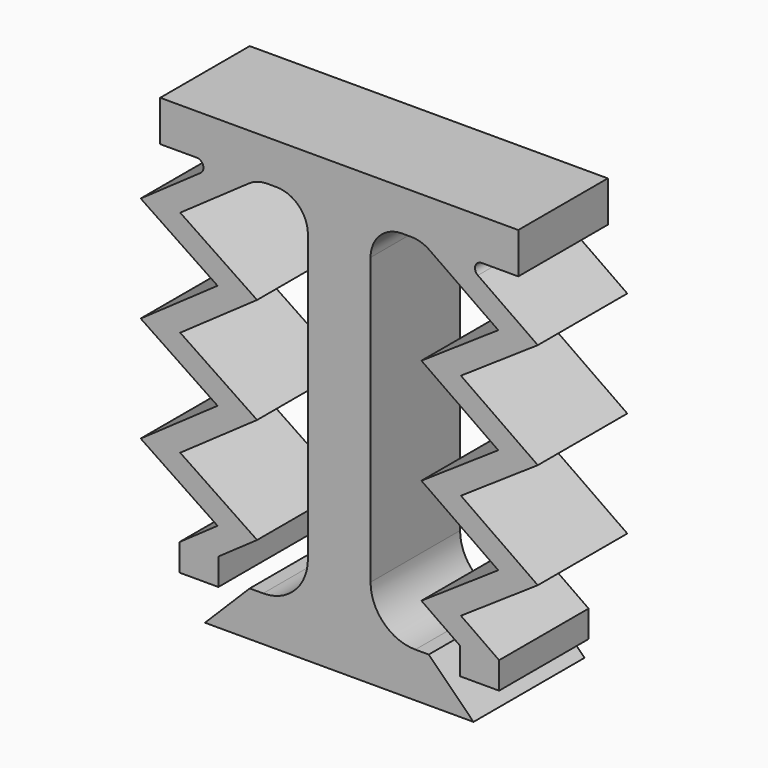
from build123d import *

# Parameters (mm, degrees)
F0_W     = 0.8717233978
F0_H     = 0.6
F1_DEPTH = 2.5
F2_DEPTH = 0.6
F4_SIZE  = 0.59999
F5_R     = 0.7
F6_R     = 1
F7_R     = 0.15


# Not quite as in the source:
# - a fillet or chamfer is up to 0.001 mm smaller than in the source, because OpenCascade refuses the exact size


with BuildPart() as f1:
    # F0 (on Front) → F1 (new body)
    with BuildSketch(Plane.XZ):
        Polygon((0, 1), (0, 0), (3, 0), (2, 1), (0.7, 1), align=None)
        Polygon((2.7075850967, 9.087372576), (1.8358616989, 9.087372576), (3.5531366706, 7.8849236956), (1.8358616989, 6.7266071015), (3.5531366706, 5.5241582211), (1.8358616989, 4.365841627), (3.5531366706, 3.1633927466), (1.8358616989, 2.0050761525), (2.7, 1.4), (3.5717233978, 1.4), (2.7185867272, 1.9973727279), (4.4358616989, 3.155689322), (2.7185867272, 4.3581382024), (4.4358616989, 5.5164547965), (2.7185867272, 6.7189036769), (4.4358616989, 7.877220271), align=None)
        with Locations((3.1358616989, 1.1)):
            Rectangle(F0_W, F0_H)
        Polygon((0, 9), (0, 1), (0.7, 1), (0.7, 9.087372576), (1.8358616989, 9.087372576), (2.7075850967, 9.087372576), (4, 9.087372576), (4, 10), (0, 10), align=None)
    extrude(amount=F1_DEPTH)

    # F0 (on Front) → F2 (join)
    with BuildSketch(Plane.XZ):
        Polygon((0, 1), (0, 0), (3, 0), (2, 1), (0.7, 1), align=None)
    extrude(amount=-F2_DEPTH)

    # F3: F1 across face


with BuildPart() as f1_1:
    add(f1.part)
    add(f1.part.mirror(Plane(origin=(0, -1.213671875, 4.89453125), x_dir=(0, -1, 0), z_dir=(-1, 0, 0))))

    # F4 (size 0.6 in the source; OpenCascade refuses exactly that, so slightly less here)
    f4_edges = [f1_1.edges().sort_by_distance(p)[0] for p in [
        (0, 0.6, 1),
    ]]
    chamfer(f4_edges, length=F4_SIZE)

    # F5
    f5_edges = [f1_1.edges().sort_by_distance(p)[0] for p in [
        (0.7, -1.25, 9.087373),
        (-0.7, -1.25, 9.087373),
        (1.835862, -1.25, 9.087373),
        (-1.835862, -1.25, 9.087373),
    ]]
    fillet(f5_edges, radius=F5_R)

    # F6
    f6_edges = [f1_1.edges().sort_by_distance(p)[0] for p in [
        (0.7, -1.25, 1),
        (-0.7, -1.25, 1),
    ]]
    fillet(f6_edges, radius=F6_R)

    # F7
    f7_edges = [f1_1.edges().sort_by_distance(p)[0] for p in [
        (2.707585, -1.25, 9.087373),
        (-2.707585, -1.25, 9.087373),
    ]]
    fillet(f7_edges, radius=F7_R)


solid = f1_1.part
